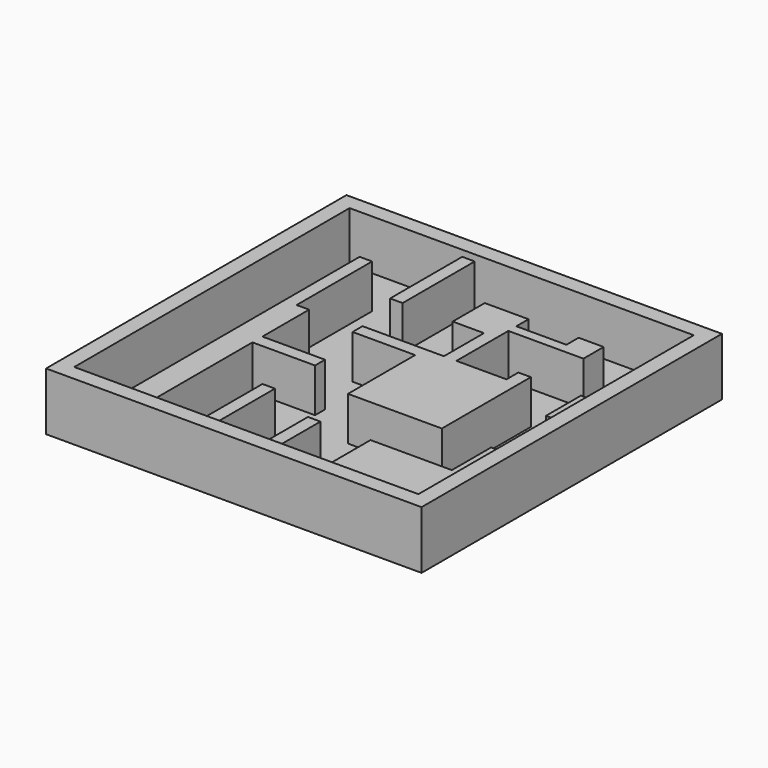
from build123d import *

# Parameters (mm, degrees)
F0_W     = 38.1
F0_H     = 38.1
F1_DEPTH = 0.79375
F2_W     = 38.1
F2_H     = 38.1
F2_W_2   = 34.925
F2_H_2   = 34.925
F3_DEPTH = 5.08
F4_W     = 1.27
F4_H     = 4.4380559438
F5_DEPTH = 4.445
F4_H_2   = 7.9962998058
F4_H_3   = 5.8306083127
F4_H_4   = 4.9851979129
F4_H_5   = 9.1487001942
F6_DEPTH = 4.445
F4_R     = 1.27
F7_DEPTH = 0.396875
F8_DEPTH = 0.396875


# Not quite as in the source:
# - a feature names something its author has since deleted; it is built from what else it names


with BuildPart() as f1:
    # F0 (on Top) → F1 (new body)
    with BuildSketch(Plane.XY):
        with Locations((-0.0411514193, 3.4528287099)):
            Rectangle(F0_W, F0_H)
    extrude(amount=F1_DEPTH)

    # F2 (on face) → F3 (join)
    with BuildSketch(Plane.XY.offset(0.79375)):
        with Locations((-0.0411514193, 3.4528287099)):
            Rectangle(F2_W, F2_H)
        with Locations((-0.0411514193, 3.4528287099)):
            Rectangle(F2_W_2, F2_H_2, mode=Mode.SUBTRACT)
    extrude(amount=F3_DEPTH)

    # F4 (on face) → F5 (join)
    with BuildSketch(Plane.XY.offset(0.79375)):
        Polygon((3.4513485807, 6.6866285157), (-4.8036514193, 6.6866285157), (-4.8036514193, 5.4166285157), (1.5463485807, 5.4166285157), (1.5463485807, -3.0990629774), (11.0713485807, -3.0990629774), (11.0713485807, 5.1481691189), (11.0713485807, 5.4166285157), (11.0713485807, 8.1909499449), (9.8013485807, 8.1909499449), (9.8013485807, 6.6866285157), (4.7213485807, 6.6866285157), (4.7213485807, 13.2709499449), (12.3413485807, 13.2709499449), (12.3413485807, 14.2892440781), (12.3413485807, 15.8353287099), (9.8013485807, 15.8353287099), (9.8013485807, 14.2892440781), (4.7213485807, 14.2892440781), (4.7213485807, 15.8353287099), (3.4513485807, 15.8353287099), (1.5463485807, 15.8353287099), (0.2763485807, 15.8353287099), (0.2763485807, 11.7666285157), (1.5463485807, 11.7666285157), (3.4513485807, 11.7666285157), align=None)
        with Locations((16.7863485807, 5.971921973)):
            Rectangle(F4_W, F4_H)
    extrude(amount=F5_DEPTH)

    # F4 (on face) → F6 (join)
    with BuildSketch(Plane.XY.offset(0.79375)):
        Polygon((-11.1536514193, 15.8353287099), (-12.4236514193, 15.8353287099), (-12.4236514193, -14.0096712901), (-9.8836514193, -14.0096712901), (-9.8836514193, -0.9333714843), (-3.5336514193, -0.9333714843), (-3.5336514193, 0.3366285157), (-9.8836514193, 0.3366285157), (-9.8836514193, 6.2576471828), (-11.1536514193, 6.2576471828), align=None)
        with Locations((-4.1686514193, -10.0115213872)):
            Rectangle(F4_W, F4_H_2)
        with Locations((2.1813485807, -11.0943671338)):
            Rectangle(F4_W, F4_H_3)
        Polygon((7.8963485807, -8.1790629774), (7.8963485807, -14.0096712901), (17.4213485807, -14.0096712901), (17.4213485807, -8.1790629774), (16.1513485807, -8.1790629774), align=None)
        with Locations((16.7863485807, -5.686464021)):
            Rectangle(F4_W, F4_H_4)
        with Locations((-5.4386514193, 16.3409786128)):
            Rectangle(F4_W, F4_H_5)
    extrude(amount=F6_DEPTH)

    # F4 (on face) → F7 (cut)
    with BuildSketch(Plane.XY.offset(0.79375)):
        with Locations((-14.9636514193, -10.9013672918)):
            Circle(F4_R)
    extrude(amount=-F7_DEPTH, mode=Mode.SUBTRACT)

    # F4 (on face) → F8 (cut)
    with BuildSketch(Plane.XY.offset(0.79375)):
        with Locations((14.2290396616, 1.2073169928)):
            Circle(F4_R)
    extrude(amount=-F8_DEPTH, mode=Mode.SUBTRACT)


solid = f1.part
